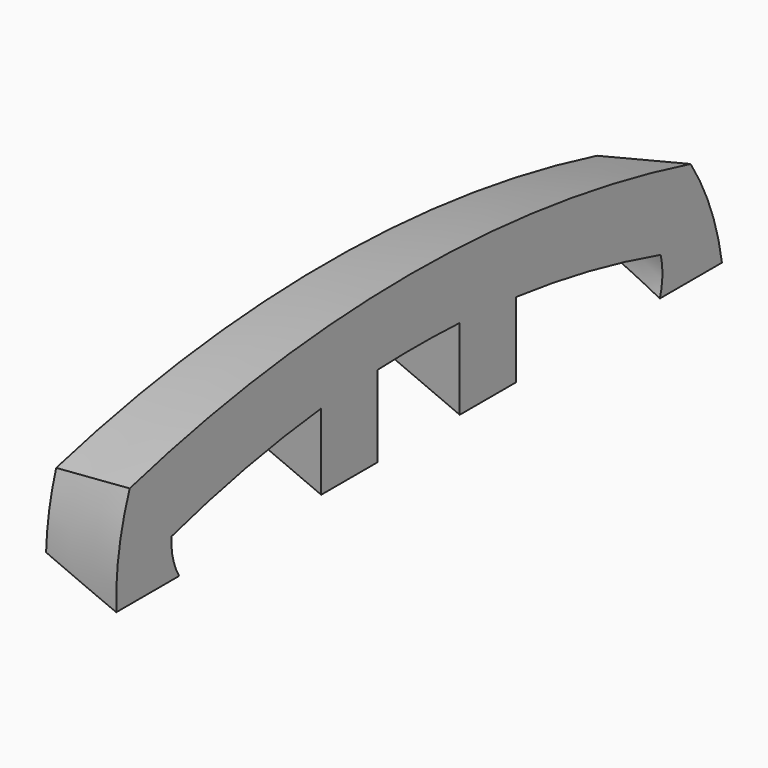
from build123d import *

# Parameters (mm, degrees)
F1_DEPTH               = 30.988
DRAFT_F1_DRAFTED_ANGLE = -12


# Not quite as in the source:
# - an extrude with a draft is written as a straight extrude whose walls are then drafted


with BuildPart() as f1:
    # F0 (on Right) → F1 (new body)
    with BuildSketch(Plane.YZ):
        with BuildLine():
            ThreePointArc((131.1102904719, -50.7162257864), (126.8298658737, -37.6063443921), (120.573348506, -25.3162257864))
            ThreePointArc((120.573348506, -25.3162257864), (-3.3422383084, -9.5432336119), (-127.2578251229, -25.3162257864))
            ThreePointArc((-127.2578251229, -25.3162257864), (-130.4972627746, -37.8474392654), (-131.8827594487, -50.7162257864))
            Line((-131.8827594487, -50.7162257864), (-119.1827594487, -50.7162257864))
            ThreePointArc((-119.1827594487, -50.7162257864), (-119.8242397153, -44.3662257864), (-119.1827594487, -38.0162257864))
            ThreePointArc((-119.1827594487, -38.0162257864), (-78.9628617731, -28.1642639268), (-37.9553229219, -22.4124747376))
            Line((-37.9553229219, -22.4124747376), (-37.9553229219, -50.9719625126))
            Line((-37.9553229219, -50.9719625126), (-25.2553229219, -50.9719625126))
            Line((-25.2553229219, -50.9719625126), (-25.2553229219, -21.4784417543))
            ThreePointArc((-25.2553229219, -21.4784417543), (0.1478038317, -20.7932458573), (25.5446770781, -21.6804727631))
            Line((25.5446770781, -21.6804727631), (25.5446770781, -50.9719744948))
            Line((25.5446770781, -50.9719744948), (38.2446770781, -50.9719744948))
            Line((38.2446770781, -50.9719744948), (38.2446770781, -22.7162511568))
            ThreePointArc((38.2446770781, -22.7162511568), (77.5990810054, -28.4763350384), (116.2117493839, -38.0162257864))
            ThreePointArc((116.2117493839, -38.0162257864), (117.9622425481, -44.2534903779), (118.4102904719, -50.7162257864))
            Line((118.4102904719, -50.7162257864), (131.1102904719, -50.7162257864))
        make_face()
    extrude(amount=F1_DEPTH)

    # draft_F1_drafted
    draft_f1_drafted_walls = [f1.faces().sort_by_distance(p)[0] for p in [
        (20.6586666667, 77.5990810054, -28.4763350384),
        (20.6586666667, 117.9622425481, -44.2534903779),
        (20.6586666667, 124.7602904719, -50.7162257864),
        (20.6586666667, 126.8298658737, -37.6063443921),
        (20.6586666667, -3.3422383084, -9.5432336119),
        (20.6586666667, -130.4972627746, -37.8474392654),
        (20.6586666667, -125.5327594487, -50.7162257864),
        (20.6586666667, -119.8242397153, -44.3662257864),
        (20.6586666667, -78.9628617731, -28.1642639268),
        (20.6586666667, -37.9553229219, -36.6922186251),
        (20.6586666667, -31.6053229219, -50.9719625126),
        (20.6586666667, -25.2553229219, -36.2252021334),
        (20.6586666667, 0.1478038317, -20.7932458573),
        (20.6586666667, 25.5446770781, -36.326223629),
        (20.6586666667, 31.8946770781, -50.9719744948),
        (20.6586666667, 38.2446770781, -36.8441128258),
    ]]
    draft(draft_f1_drafted_walls, neutral_plane=Plane.YZ, angle=DRAFT_F1_DRAFTED_ANGLE)


solid = f1.part
